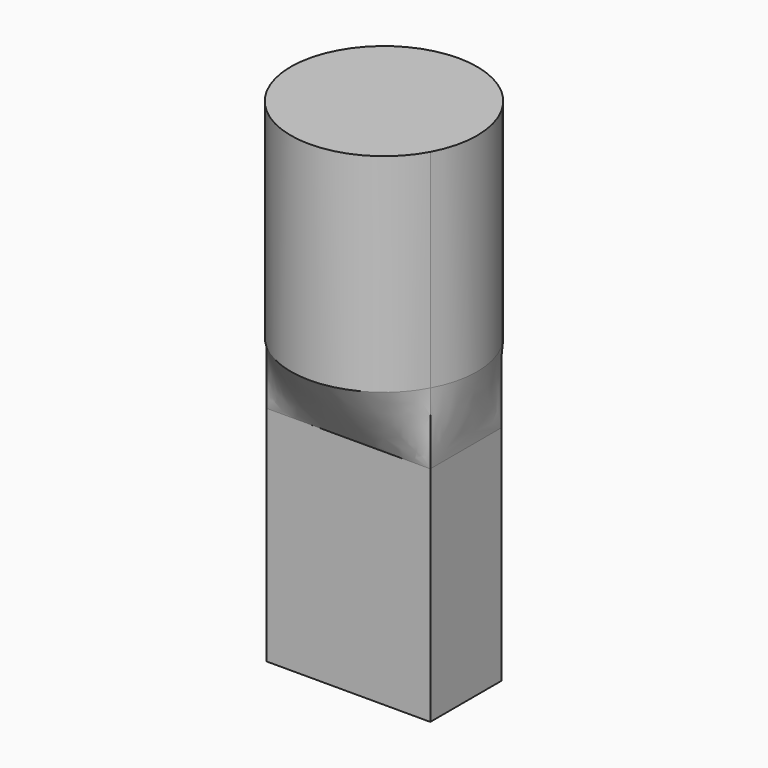
from build123d import *

# Parameters (mm, degrees)
F0_W      = 18.5
F0_H      = 5
F1_DEPTH  = 3
F4_DEPTH  = 58.4
F1_FACE_W = 46
F1_FACE_H = 25
F6_DEPTH  = 59.6


with BuildPart() as f1:
    # F0 (on Top) → F1 (new body)
    with BuildSketch(Plane.XY):
        Polygon((-56.2144573331, 13.5414201766), (-10.2144573331, 13.5414201766), (-10.2144573331, 38.5414201766), (-23.9644573331, 38.5414201766), (-23.9644573331, 33.5414201766), (-15.2144573331, 33.5414201766), (-15.2144573331, 18.5414201766), (-51.2144573331, 18.5414201766), (-51.2144573331, 33.5414201766), (-42.4644573331, 33.5414201766), (-42.4644573331, 38.5414201766), (-56.2144573331, 38.5414201766), align=None)
        with Locations((-33.2144573331, 36.0414201766)):
            Rectangle(F0_W, F0_H)
        Polygon((-15.2144573331, 33.5414201766), (-23.9644573331, 33.5414201766), (-42.4644573331, 33.5414201766), (-51.2144573331, 33.5414201766), (-51.2144573331, 18.5414201766), (-15.2144573331, 18.5414201766), align=None)
    extrude(amount=F1_DEPTH)

    # F1_face (on face) → F5 section 0
    with BuildSketch(Plane(origin=(-33.2144573331, 26.0414201766, 3), x_dir=(1, 0, 0), z_dir=(0, 0, 1))):
        Rectangle(F1_FACE_W, F1_FACE_H)
    # F3 (on offset) → F5 section 1
    with BuildSketch(Plane.XY.offset(23)):
        with BuildLine():
            ThreePointArc((-10.2144573331, 38.5414201766), (-33.2144573331, 52.218700402), (-56.2144573331, 38.5414201766))
            ThreePointArc((-56.2144573331, 38.5414201766), (-59.3917375585, 26.0414201766), (-56.2144573331, 13.5414201766))
            ThreePointArc((-56.2144573331, 13.5414201766), (-33.2144573331, -0.1358600488), (-10.2144573331, 13.5414201766))
            ThreePointArc((-10.2144573331, 13.5414201766), (-7.0371771077, 26.0414201766), (-10.2144573331, 38.5414201766))
        make_face()
    loft()

    # F0 (on Top) → F6 (join)
    with BuildSketch(Plane.XY):
        Polygon((-56.2144573331, 13.5414201766), (-10.2144573331, 13.5414201766), (-10.2144573331, 38.5414201766), (-23.9644573331, 38.5414201766), (-23.9644573331, 33.5414201766), (-15.2144573331, 33.5414201766), (-15.2144573331, 18.5414201766), (-51.2144573331, 18.5414201766), (-51.2144573331, 33.5414201766), (-42.4644573331, 33.5414201766), (-42.4644573331, 38.5414201766), (-56.2144573331, 38.5414201766), align=None)
    extrude(amount=-F6_DEPTH)


with BuildPart() as f4:
    # F3 (on offset) → F4 (new body)
    with BuildSketch(Plane.XY.offset(23)):
        with BuildLine():
            ThreePointArc((-10.2144573331, 38.5414201766), (-33.2144573331, 52.218700402), (-56.2144573331, 38.5414201766))
            ThreePointArc((-56.2144573331, 38.5414201766), (-59.3917375585, 26.0414201766), (-56.2144573331, 13.5414201766))
            ThreePointArc((-56.2144573331, 13.5414201766), (-33.2144573331, -0.1358600488), (-10.2144573331, 13.5414201766))
            ThreePointArc((-10.2144573331, 13.5414201766), (-7.0371771077, 26.0414201766), (-10.2144573331, 38.5414201766))
        make_face()
    extrude(amount=F4_DEPTH)


solid = Compound([f1.part, f4.part])
